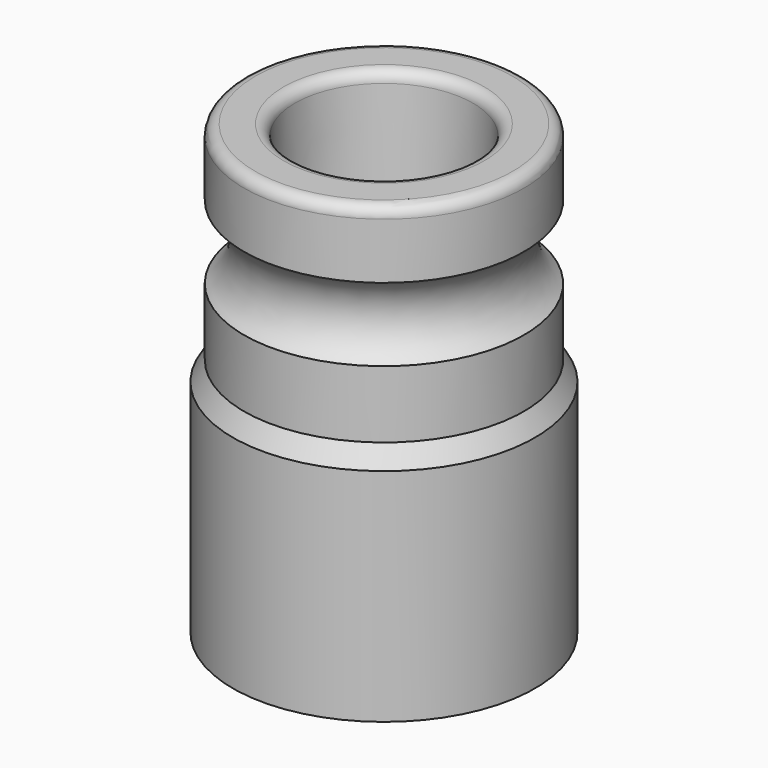
from build123d import *

# Parameters (mm, degrees)
F2_R     = 2
F3_R     = 18
F3_R_2   = 14
F4_DEPTH = 30


# Not quite as in the source:
# - a feature names something its author has since deleted; it is built from what else it names


with BuildPart() as f1:
    # F0 (on Front) → F1 (revolve)
    with BuildSketch(Plane.XZ):
        with BuildLine():
            Line((-14, -9.4360596032), (-16, 40.5639403968))
            Line((-16, 40.5639403968), (-25, 40.5639403968))
            Line((-25, 40.5639403968), (-25, 28.5639403968))
            ThreePointArc((-25, 28.5639403968), (-21.593316446, 22.014021006), (-25, 15.4641016151))
            Line((-25, 15.4641016151), (-25, 3.4641016151))
            Line((-25, 3.4641016151), (-27, 0))
            Line((-27, 0), (-27, -39.4360596032))
            Line((-27, -39.4360596032), (-18, -39.4360596032))
            Line((-18, -39.4360596032), (-14, -39.4360596032))
            Line((-14, -39.4360596032), (-14, -9.4360596032))
        make_face()
    revolve(axis=Axis((0, 0, -1.7232764512), (0, 0, -1)))

    # F2
    f2_edges = [f1.edges().sort_by_distance(p)[0] for p in [
        (16, 0, 40.56394),
        (25, 0, 40.56394),
    ]]
    fillet(f2_edges, radius=F2_R)

    # F3 (on face) → F4 (cut)
    with BuildSketch(Plane(origin=(0, 0, -39.4360596032), x_dir=(1, 0, 0), z_dir=(0, 0, -1))):
        Circle(F3_R)
        Circle(F3_R_2, mode=Mode.SUBTRACT)
    extrude(amount=-F4_DEPTH, mode=Mode.SUBTRACT)


solid = f1.part
